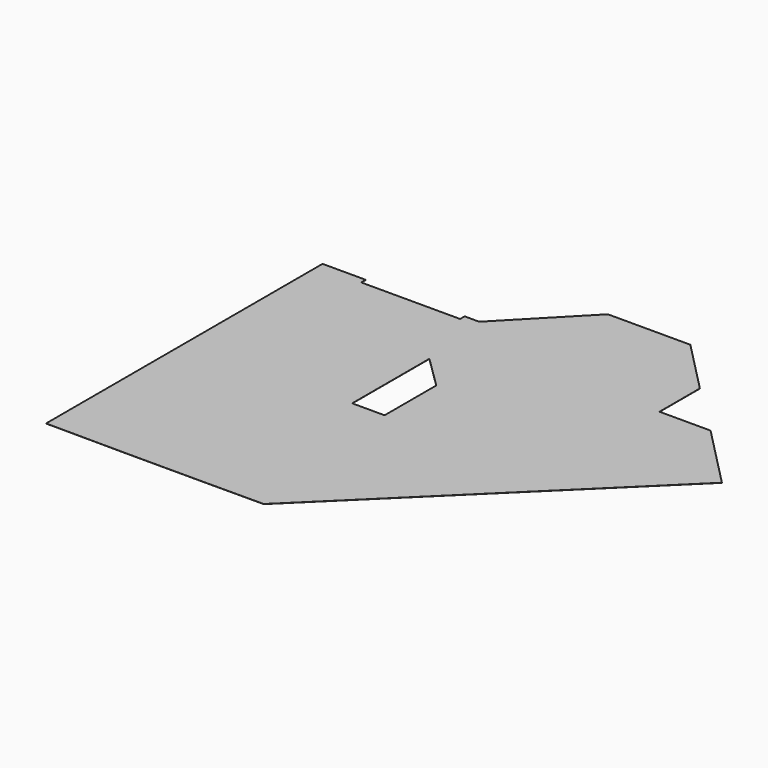
from build123d import *

# Parameters (mm, degrees)
F4_DEPTH = 3.048


# Not quite as in the source:
# - the program builds the solid bodies; features that only make, move or delete a surface that nothing else refers to are left out


with BuildPart() as f4:
    # F0 (on Top) → F4 (new body)
    with BuildSketch(Plane.XY):
        Polygon((-859.3434095383, 2249.2264169165), (-1783.9930057526, 2249.2264169165), (-1783.9930057526, -1707.3482275009), (619.3107366562, -1707.3482275009), (619.3107366562, -2341.3591384888), (0, -2341.3591384888), (-1783.9930057526, -2341.3591384888), (-1783.9930057526, -5145.3490257263), (0, -5154.3831825256), (1534.4239473343, -5154.3831825256), (2877.5852176544, -5150.4210421951), (3421.4589595795, -4617.690990831), (6357.0975280814, -1742.2021322423), (8374.4828170111, 233.8479796617), (7047.7240208756, 1588.3600242488), (5956.0112953186, 1588.3600242488), (5956.0112953186, 2667.5424575806), (4844.0600873968, 3802.7535513455), (3078.5310268402, 3802.7535513455), (1568.8069942474, 2249.2264169165), (1257.5402259827, 2249.2264169165), (1257.5402259827, 2127.9256343842), (-859.3434095383, 2127.9256343842), align=None)
        Polygon((1756.28054142, -1382.1313381195), (1756.28054142, 681.4878258383), (2449.0561485291, 0), (2449.0561485291, -1382.1313381195), align=None, mode=Mode.SUBTRACT)
        Polygon((619.3107366562, -1707.3482275009), (-1783.9930057526, -1707.3482275009), (-1783.9930057526, -2341.3591384888), (0, -2341.3591384888), (619.3107366562, -2341.3591384888), align=None)
    extrude(amount=-F4_DEPTH)


solid = f4.part
